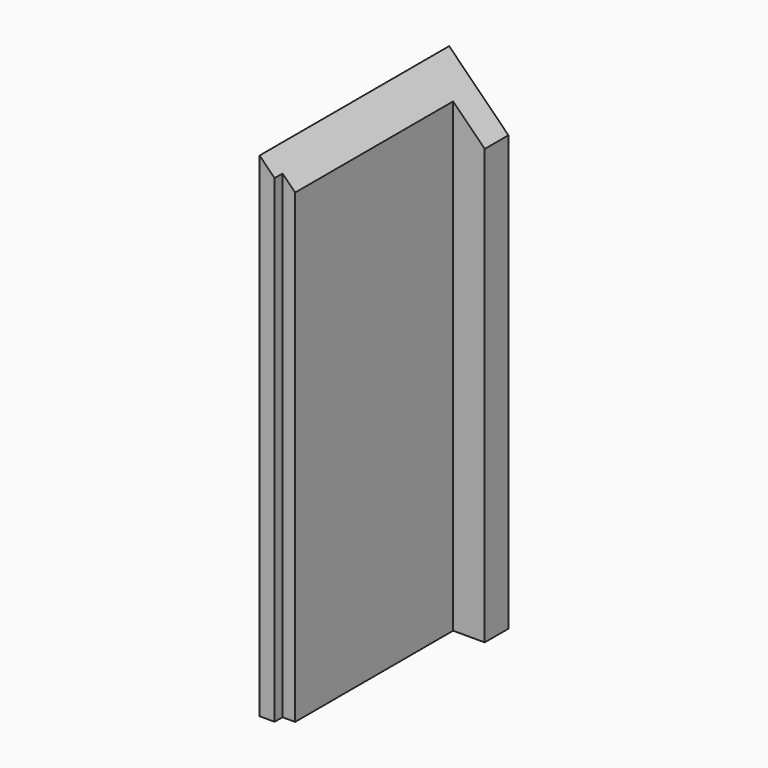
from build123d import *

# Parameters (mm, degrees)
F1_DEPTH = 76.2
F2_W     = 153.924
F2_H     = 153.924
F3_DEPTH = 3.175
F4_W     = 149.86
F4_H     = 149.86
F5_DEPTH = 63.5
F7_DEPTH = 76.201


# Not quite as in the source:
# - a feature names something its author has since deleted; it is built from what else it names


with BuildPart() as f1:
    # F0 (on Front) → F1 (new body)
    with BuildSketch(Plane.XZ):
        Polygon((0, 139.7), (0, 158.75), (-158.75, 158.75), (-158.75, 0), (-139.7, 0), (-139.7, 139.7), align=None)
    extrude(amount=F1_DEPTH)

    # F2 (on face) → F3 (cut)
    with BuildSketch(Plane.XZ.offset(76.2)):
        with Locations((-76.962, 76.962)):
            Rectangle(F2_W, F2_H)
    extrude(amount=-F3_DEPTH, mode=Mode.SUBTRACT)

    # F4 (on face) → F5 (cut)
    with BuildSketch(Plane.XZ.offset(73.025)):
        with Locations((-74.93, 74.93)):
            Rectangle(F4_W, F4_H)
    extrude(amount=-F5_DEPTH, mode=Mode.SUBTRACT)

    # F6 (on face) → F7 (cut, through all)
    with BuildSketch(Plane.XZ.offset(76.2)):
        Polygon((0, 158.75), (-158.75, 158.75), (-139.7, 139.7), (0, 139.7), align=None)
    extrude(amount=-F7_DEPTH, mode=Mode.SUBTRACT)


solid = f1.part
